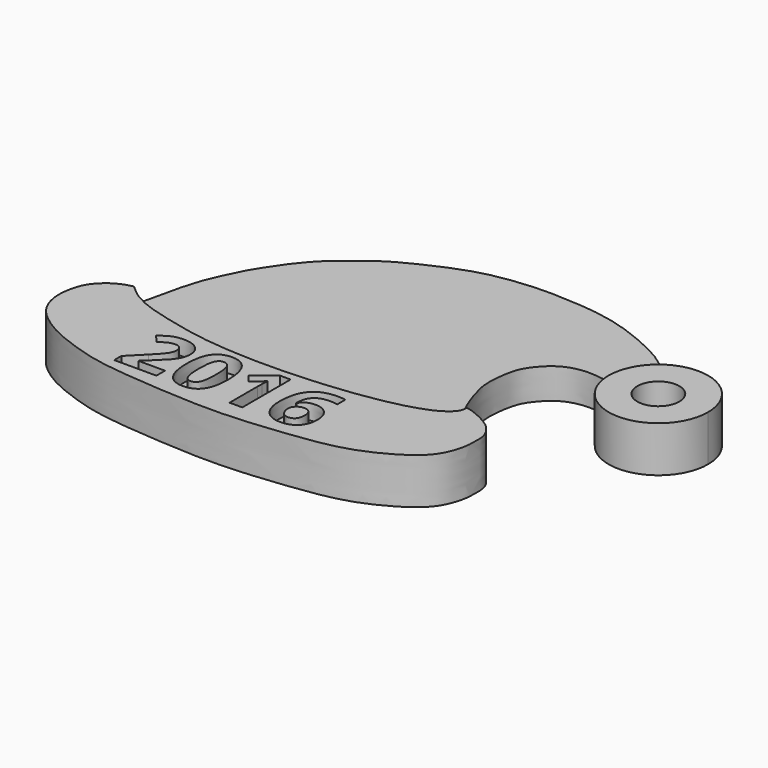
from build123d import *

# Parameters (mm, degrees)
F1_DEPTH     = 6
F2_DEPTH     = 4
F3_TEXT_SIZE = 11.0611642918
F4_DEPTH     = 2
F5_D         = 5.5


# Not quite as in the source:
# - Text() gives the source's letters only with a copy of the font that has no kerning and outlines rounded to 1/6400 em; it was checked with that copy


with BuildPart() as f1:
    # F0 (on Top) → F1 (new body)
    with BuildSketch(Plane.XY):
        with BuildLine():
            add(Edge.make_bspline(
                [(53.1659834087, 19.3741284311), (53.1749584793, 19.2385227848), (53.1938676928, 18.9528207302), (53.0288648596, 18.4535148322), (52.5810572286, 17.8423255035), (51.7478920389, 17.2350787963), (50.8023592404, 16.7041358741), (48.9706128006, 16.0237827147), (46.5317488574, 15.3871689237), (43.321534276, 14.8074780368), (38.8996397958, 14.253574786), (32.8898195743, 13.9174039656), (27.4957595748, 13.9903860884), (21.8776883799, 14.4505462963), (16.331901366, 15.8034770244), (13.4872978312, 16.638266812), (11.6771725948, 17.5977483006), (10.8384111491, 18.2221045397), (10.2105676248, 18.7780194086), (9.8807457834, 19.0700553358)],
                knots=[0, 0, 0, 0, 0.0246896725, 0.0520176729, 0.0853119721, 0.1239893005, 0.163998025, 0.2171478276, 0.2784723648, 0.3474874404, 0.4290942858, 0.5237640734, 0.6135099671, 0.7056705893, 0.7976221084, 0.8642087416, 0.9175556956, 0.9566899534, 1, 1, 1, 1], degree=3))
            add(Edge.make_bspline(
                [(9.8807457834, 19.0700553358), (9.5790048058, 19.0123995211), (8.8797183573, 18.8787818395), (7.3384309321, 18.1061638348), (6.0713932407, 16.8329557271), (5.3819524595, 15.5936665561), (4.9234718471, 13.5628780528), (5.0246391758, 11.7815321357), (5.5110811339, 10.262907092), (6.4468032858, 8.8650728758), (8.0481787943, 7.5335335521), (10.4236231769, 6.0545879757), (14.9341820916, 4.4322727035), (18.8366396402, 3.560822115), (25.9126344067, 2.9689952728), (33.7972842815, 2.5271342472), (41.7140079212, 3.2903301318), (48.4348492596, 4.1875146189), (53.0384935079, 6.1022723996), (57.443198723, 8.9271731103), (58.4650590276, 12.5997528867), (58.4617183834, 13.8814547813), (58.5619519632, 15.8034404067), (57.3180184428, 17.4443328454), (56.2226791624, 18.1489288902), (55.2200259439, 18.6704053539), (54.0831687362, 19.1680737245), (53.4571185141, 19.3087220657), (53.1659834087, 19.3741284311)],
                knots=[0, 0, 0, 0, 0.0231968649, 0.0537588676, 0.0848890686, 0.11262029, 0.1459904639, 0.1772917395, 0.2063789139, 0.2362596658, 0.2693461425, 0.3085973137, 0.3591287685, 0.4063213143, 0.4678490776, 0.5343767039, 0.6005913899, 0.6609598979, 0.7131929568, 0.7659532166, 0.8094562635, 0.835919713, 0.8673202274, 0.9002340095, 0.9267603834, 0.9515234543, 0.9774567219, 1, 1, 1, 1], degree=3))
        make_face()
    extrude(amount=F1_DEPTH)

    # F3 (on face) → F4 (cut)
    with BuildSketch(Plane.XY.offset(6)):
        with Locations((18.0211216211, 5.1062437706)):
            Text('2016', F3_TEXT_SIZE, font='Open Sans', font_style=FontStyle.BOLD, text_align=(TextAlign.LEFT, TextAlign.BOTTOM))
    extrude(amount=-F4_DEPTH, mode=Mode.SUBTRACT)


with BuildPart() as f1b:
    # F0 (on Top) → F1, piece 2 (new body)
    with BuildSketch(Plane.XY):
        with BuildLine():
            ThreePointArc((73.0211975574, 33.986415714), (69.6982460785, 39.6570737618), (63.1269321128, 39.5297867183))
            ThreePointArc((63.1269321128, 39.5297867183), (61.2534935998, 37.7944723069), (60.1931003152, 35.4714023445))
            ThreePointArc((60.1931003152, 35.4714023445), (65.7737459117, 27.5295344206), (73.0211975574, 33.986415714))
        make_face()
    extrude(amount=F1_DEPTH)

    # F5 (through all)
    with Locations(Plane(origin=(0, 0, 0), x_dir=(1, 0, 0), z_dir=(0, 0, -1))):
        with Locations((66.5211975574, -33.986415714)):
            Hole(F5_D / 2)


with BuildPart() as f2:
    # F0 (on Top) → F2 (new body)
    with BuildSketch(Plane.XY):
        with BuildLine():
            add(Edge.make_bspline(
                [(9.8807457834, 19.0700553358), (9.986807713, 19.1043521739), (10.2468032281, 19.1884259236), (10.2376465381, 19.9560301125), (10.3750404592, 20.5969404825), (10.6134825078, 21.5967116392), (10.8047164972, 22.4395111402), (11.1055837131, 23.8101196295), (11.4285461738, 25.2840575697), (12.1266725345, 27.5276512586), (12.5915433527, 28.6545901036), (14.1325547135, 31.9703995433), (14.9896103515, 33.2746977002), (16.8551867231, 36.2375260881), (19.5047372397, 39.0866311593), (20.7156726948, 39.8626807573), (23.2511543825, 42.138924919), (26.9624842226, 44.0612179184), (30.0194301168, 45.4454137246), (33.2022227196, 46.6052026227), (36.7506245854, 47.2949212296), (40.8444831345, 47.5776738728), (43.0161343811, 47.4540288122), (47.1447492529, 47.2992174662), (51.3635120206, 46.4658086213), (54.9728834904, 45.0794112917), (58.5391989557, 43.4390704141), (61.0456754321, 41.4664908905), (62.4469246688, 40.1635174739), (63.1269321128, 39.5297867183)],
                knots=[0, 0, 0, 0, 0.0135348224, 0.0331806331, 0.0532606826, 0.077024715, 0.0995271665, 0.1271774724, 0.157445684, 0.1930606291, 0.2210500927, 0.2654908928, 0.2965244356, 0.3410924541, 0.3879283757, 0.4165201432, 0.4595535072, 0.509067291, 0.5528718477, 0.5962172136, 0.6423375687, 0.6899841916, 0.7254922753, 0.773294796, 0.8233286328, 0.8703604432, 0.9174650376, 0.959985248, 1, 1, 1, 1], degree=3))
            add(Edge.make_bspline(
                [(53.1659834087, 19.3741284311), (53.1749584793, 19.2385227848), (53.1938676928, 18.9528207302), (53.0288648596, 18.4535148322), (52.5810572286, 17.8423255035), (51.7478920389, 17.2350787963), (50.8023592404, 16.7041358741), (48.9706128006, 16.0237827147), (46.5317488574, 15.3871689237), (43.321534276, 14.8074780368), (38.8996397958, 14.253574786), (32.8898195743, 13.9174039656), (27.4957595748, 13.9903860884), (21.8776883799, 14.4505462963), (16.331901366, 15.8034770244), (13.4872978312, 16.638266812), (11.6771725948, 17.5977483006), (10.8384111491, 18.2221045397), (10.2105676248, 18.7780194086), (9.8807457834, 19.0700553358)],
                knots=[0, 0, 0, 0, 0.0246896725, 0.0520176729, 0.0853119721, 0.1239893005, 0.163998025, 0.2171478276, 0.2784723648, 0.3474874404, 0.4290942858, 0.5237640734, 0.6135099671, 0.7056705893, 0.7976221084, 0.8642087416, 0.9175556956, 0.9566899534, 1, 1, 1, 1], degree=3))
            add(Edge.make_bspline(
                [(53.1659834087, 19.3741284311), (53.014839423, 19.3479069005), (52.6336862925, 19.2817817523), (51.7117738005, 20.0689683228), (50.8871925601, 21.8507243444), (50.1447937814, 23.3314846716), (49.5516680695, 25.1517148606), (49.0007435806, 26.9886881285), (48.9578991516, 29.0440585901), (49.2688787604, 31.0847183806), (49.7403096111, 32.7657024138), (51.306529216, 34.6866632136), (52.8770191702, 35.7623316837), (54.7547447354, 36.2370957493), (56.4654795943, 36.2336421908), (58.5685635355, 35.9112418286), (59.6708832346, 35.6127365038), (60.1931003152, 35.4714023445)],
                knots=[0, 0, 0, 0, 0.0348414979, 0.0878792517, 0.1592994188, 0.2252643106, 0.2947253614, 0.3648955341, 0.4374272032, 0.5096611582, 0.5765129773, 0.6550338768, 0.7251960114, 0.7941541706, 0.8607690561, 0.9343007554, 1, 1, 1, 1], degree=3))
            ThreePointArc((60.1931003152, 35.4714023445), (61.2534935998, 37.7944723069), (63.1269321128, 39.5297867183))
        make_face()
    extrude(amount=F2_DEPTH)


solid = Compound([f1.part, f1b.part, f2.part])
